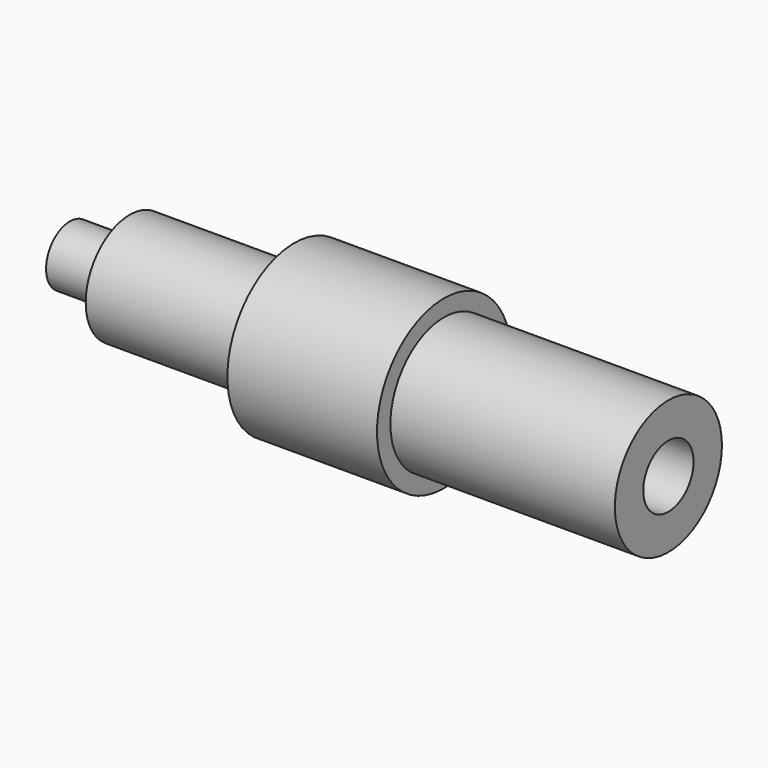
from build123d import *

# Parameters (mm, degrees)
F0_R      = 7.1015967563
F1_DEPTH  = 12.7
F2_R      = 5.6788395521
F3_DEPTH  = 19.05
F4_R      = 4.6676560737
F5_DEPTH  = 13.97
F6_R      = 2.5243045871
F7_DEPTH  = 5.08
F8_R      = 2.6650653171
F9_DEPTH  = 43.18
F10_R     = 0.7037770969
F11_DEPTH = 25.4
F12_SIZE  = 0.381


# Not quite as in the source:
# - the program builds the solid bodies; features that only make, move or delete a surface that nothing else refers to are left out


with BuildPart() as f1:
    # F0 (on Right) → F1 (new body)
    with BuildSketch(Plane.YZ):
        Circle(F0_R)
    extrude(amount=F1_DEPTH)

    # F2 (on face) → F3 (join)
    with BuildSketch(Plane.YZ.offset(12.7)):
        Circle(F2_R)
    extrude(amount=F3_DEPTH)

    # F4 (on face) → F5 (join)
    with BuildSketch(Plane(origin=(0, 0, 0), x_dir=(0, -1, 0), z_dir=(-1, 0, 0))):
        Circle(F4_R)
    extrude(amount=F5_DEPTH)

    # F6 (on face) → F7 (join)
    with BuildSketch(Plane(origin=(-13.97, 0, 0), x_dir=(0, -1, 0), z_dir=(-1, 0, 0))):
        Circle(F6_R)
    extrude(amount=F7_DEPTH)

    # F8 (on face) → F9 (cut)
    with BuildSketch(Plane.YZ.offset(31.75)):
        Circle(F8_R)
    extrude(amount=-F9_DEPTH, mode=Mode.SUBTRACT)

    # F10 (on face) → F11 (cut)
    with BuildSketch(Plane(origin=(-19.05, 0, 0), x_dir=(0, -1, 0), z_dir=(-1, 0, 0))):
        Circle(F10_R)
    extrude(amount=-F11_DEPTH, mode=Mode.SUBTRACT)

    # F12
    f12_edges = [f1.edges().sort_by_distance(p)[0] for p in [
        (-11.43, 0.703777, 0),
    ]]
    chamfer(f12_edges, length=F12_SIZE)


solid = f1.part
